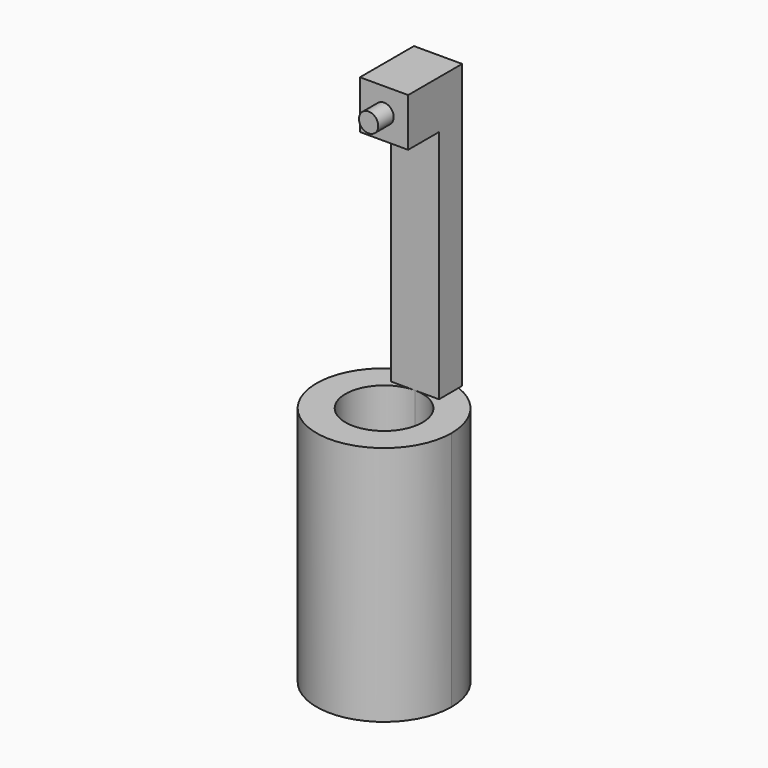
from build123d import *

# Parameters (mm, degrees)
F0_W     = 5
F0_H     = 5
F1_DEPTH = 4
F2_R     = 1
F3_DEPTH = 2
F4_W     = 5
F4_H     = 24.4
F4_H_2   = 5
F5_DEPTH = 3
F7_DEPTH = 25


with BuildPart() as f1:
    # F0 (on Front) → F1 (new body)
    with BuildSketch(Plane.XZ):
        Rectangle(F0_W, F0_H)
    extrude(amount=F1_DEPTH)

    # F2 (on face) → F3 (join)
    with BuildSketch(Plane.XZ.offset(4)):
        Circle(F2_R)
    extrude(amount=F3_DEPTH)

    # F4 (on face) → F5 (join)
    with BuildSketch(Plane(origin=(0, 0, 0), x_dir=(-1, 0, 0), z_dir=(0, 1, 0))):
        with Locations((0, -14.7)):
            Rectangle(F4_W, F4_H)
        Rectangle(F4_W, F4_H_2)
    extrude(amount=F5_DEPTH)

    # F6 (on face) → F7 (join)
    with BuildSketch(Plane(origin=(0, 0, -26.9), x_dir=(1, 0, 0), z_dir=(0, 0, -1))):
        with BuildLine():
            Line((-2.5, 0), (0, 0))
            Line((0, 0), (2.5, 0))
            Line((2.5, 0), (2.5, -2.5383484153))
            ThreePointArc((2.5, -2.5383484153), (5.7662812973, 0.0313730334), (7, 4))
            ThreePointArc((7, 4), (-3.9686269666, 9.7662812973), (-2.5, -2.5383484153))
            Line((-2.5, -2.5383484153), (-2.5, 0))
        make_face()
        with BuildLine():
            ThreePointArc((0, 0), (-2.8284271247, 6.8284271247), (4, 4))
            ThreePointArc((4, 4), (2.8284271247, 1.1715728753), (0, 0))
        make_face(mode=Mode.SUBTRACT)
        with BuildLine():
            Line((2.5, 0), (0, 0))
            Line((0, 0), (-2.5, 0))
            Line((-2.5, 0), (-2.5, -2.5383484153))
            ThreePointArc((-2.5, -2.5383484153), (-1.2711335675, -2.8836196477), (0, -3))
            ThreePointArc((0, -3), (1.2711335675, -2.8836196477), (2.5, -2.5383484153))
            Line((2.5, -2.5383484153), (2.5, 0))
        make_face()
    extrude(amount=F7_DEPTH)


solid = f1.part
